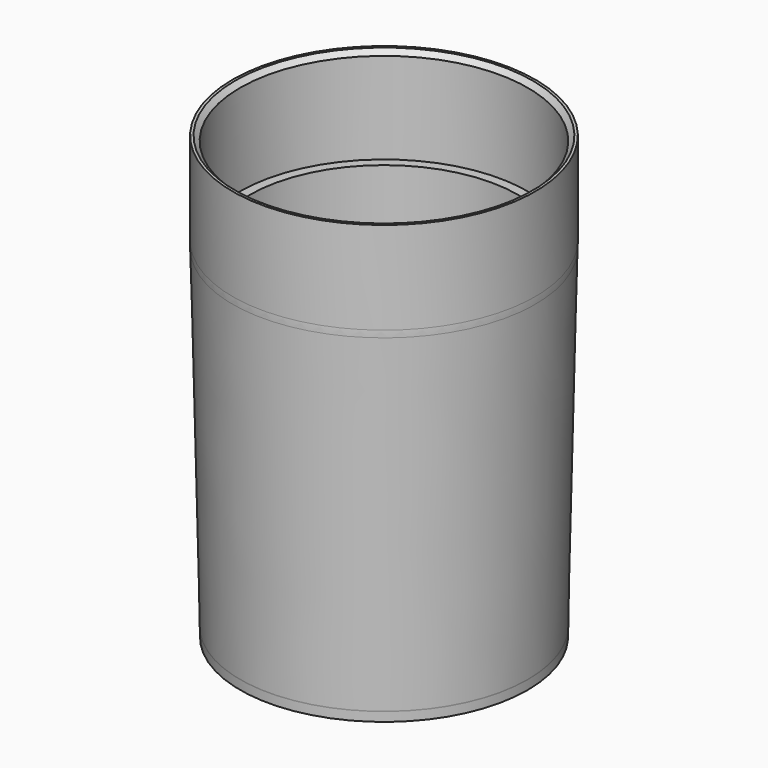
from build123d import *

# Parameters (mm, degrees)
F3_SIZE = 0.5


# Not quite as in the source:
# - a fillet or chamfer that OpenCascade refuses, or shapes differently, is made with other operations: its cross-section is extruded or revolved along the edge and cut away or added


with BuildPart() as f1:
    # F0 (on Front) → F1 (revolve)
    with BuildSketch(Plane.XZ):
        with BuildLine():
            Line((0, -1), (0, 0))
            Line((0, 0), (-13, 0))
            ThreePointArc((-13, 0), (-13.7071067812, 0.2928932188), (-14, 1))
            Line((-14, 1), (-14, 34.9983884289))
            Line((-14, 34.9983884289), (-15, 34.9983884289))
            Line((-15, 34.9983884289), (-15, 45))
            Line((-15, 45), (-15.7777419651, 45))
            Line((-15.7777419651, 45), (-15.7777419651, 34.9983884289))
            Line((-15.7777419651, 34.9983884289), (-15, 0))
            Line((-15, 0), (-14.9990128332, -0.0444225074))
            Line((-14.9990128332, -0.0444225074), (-14.9777777778, -1))
            Line((-14.9777777778, -1), (0, -1))
        make_face()
        with BuildLine():
            ThreePointArc((-15, 0), (-14.9997531778, -0.0222167373), (-14.9990128332, -0.0444225074))
            Line((-14.9990128332, -0.0444225074), (-15, 0))
        make_face()
    revolve(axis=Axis((0, 0, 35.2895334363), (0, 0, 1)))

    # F2: fillet of radius 50 on 1 edges, made by hand

    # F2_s1 → F2_t2 (revolve, cut)
    with BuildSketch(Plane.XZ):
        with BuildLine():
            ThreePointArc((-15.7658002643, 34.4430074493), (-15.7750564447, 34.9984182643), (-15.7781419651, 35.5538976338))
            Line((-15.7781419651, 35.5538976338), (-20.7783819651, 35.5538976338))
            ThreePointArc((-20.7783819651, 35.5538976338), (-20.7779819651, 35.2761430313), (-20.7779819651, 34.9983884289))
            Line((-20.7779819651, 34.9983884289), (-20.776747795, 34.8872994105))
            ThreePointArc((-20.776747795, 34.8872994105), (-20.770576994, 34.609613364), (-20.7648060942, 34.3319184309))
            Line((-20.7648060942, 34.3319184309), (-15.7658002643, 34.4430074493))
        make_face()
    revolve(axis=Axis((0, 0, 34.9983884289), (0, 0, 1)), mode=Mode.SUBTRACT)

    # F3
    f3_edges = [f1.edges().sort_by_distance(p)[0] for p in [
        (15, 0, 45),
    ]]
    chamfer(f3_edges, length=F3_SIZE)


solid = f1.part
